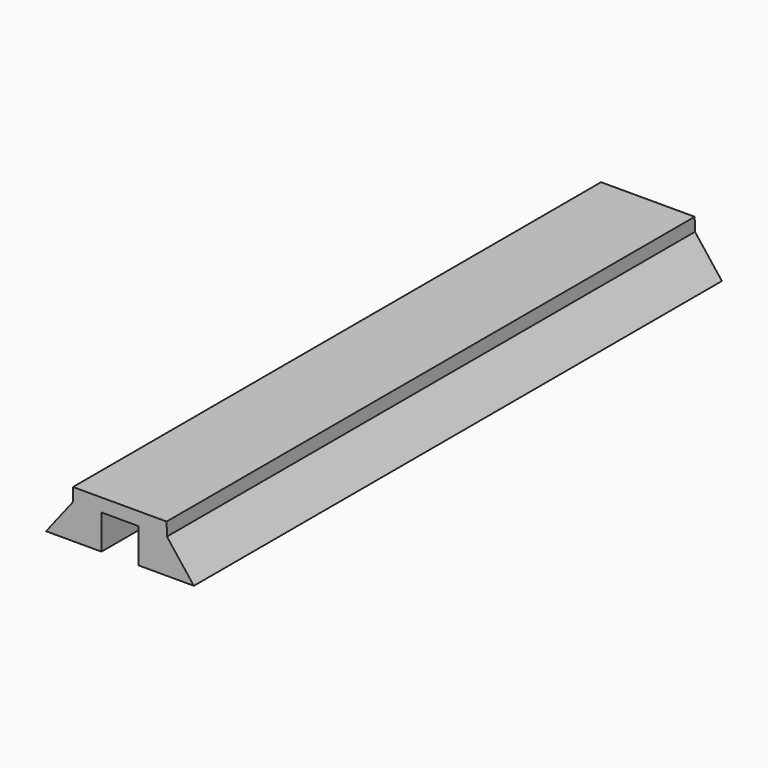
from build123d import *

# Parameters (mm, degrees)
F1_DEPTH = 400


# Not quite as in the source:
# - a feature names something its author has since deleted; it is built from what else it names


with BuildPart() as f1:
    # F0 (on Front) → F1 (new body)
    with BuildSketch(Plane.XZ):
        Polygon((11.218088679, 20.9527928382), (11.218088679, 0), (28.4624192864, 0), (44.7796396911, 0), (28.4582051874, 20.9527928382), (28.2770004123, 28.9259795099), (-28.4582051874, 28.9259795099), (-28.4582051874, 20.9527928382), (-44.7796396911, 0), (-28.4624192864, 0), (-11.218088679, 0), (-11.218088679, 20.9527928382), align=None)
    extrude(amount=-F1_DEPTH)


solid = f1.part
